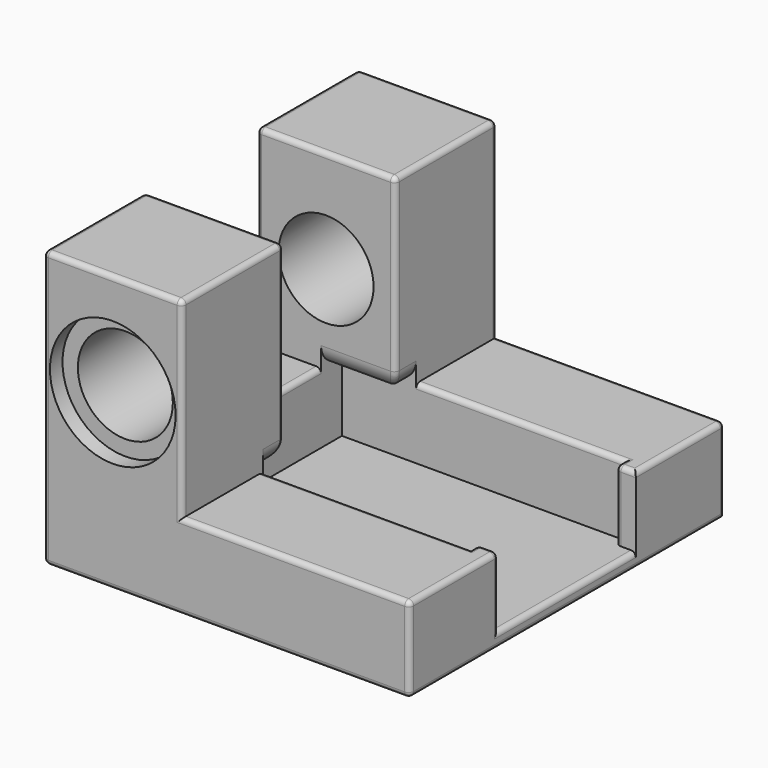
from build123d import *

# Parameters (mm, degrees)
F1_DEPTH  = 39.766
F2_R      = 4.8
F3_DEPTH  = 39.767
F2_R_2    = 6.35
F4_DEPTH  = 1.5875
F5_R      = 6.35
F6_DEPTH  = 1.5875
F7_W      = 7.5
F7_H      = 19.36
F8_DEPTH  = 7.1
F10_DEPTH = 19.3
F11_R     = 2
F12_R     = 0.5


with BuildPart() as f1:
    # F0 (on Front) → F1 (new body)
    with BuildSketch(Plane.XZ):
        Polygon((0, 27.9), (0, 0), (37, 0), (37, 8.6), (14, 8.6), (14, 27.9), align=None)
    extrude(amount=F1_DEPTH)

    # F2 (on face) → F3 (cut, through all)
    with BuildSketch(Plane.XZ.offset(39.766)):
        with Locations((7, 17.55)):
            Circle(F2_R)
    extrude(amount=-F3_DEPTH, mode=Mode.SUBTRACT)

    # F2 (on face) → F4 (cut)
    with BuildSketch(Plane.XZ.offset(39.766)):
        with Locations((7, 17.55)):
            Circle(F2_R_2)
        with Locations((7, 17.55)):
            Circle(F2_R, mode=Mode.SUBTRACT)
    extrude(amount=-F4_DEPTH, mode=Mode.SUBTRACT)

    # F5 (on face) → F6 (cut)
    with BuildSketch(Plane.XZ):
        with Locations((7, 17.55)):
            Circle(F5_R)
    extrude(amount=F6_DEPTH, mode=Mode.SUBTRACT)

    # F7 (on face) → F8 (cut)
    with BuildSketch(Plane.XY.offset(8.6)):
        with Locations((10.25, -19.883)):
            Rectangle(F7_W, F7_H)
        Polygon((37, -28.563), (37, -11.203), (35, -11.203), (35, -10.203), (14, -10.203), (14, -29.563), (35, -29.563), (35, -28.563), align=None)
    extrude(amount=-F8_DEPTH, mode=Mode.SUBTRACT)

    # F9 (on face) → F10 (cut, through all)
    with BuildSketch(Plane.XY.offset(27.9)):
        Polygon((0, -12.827), (0, -19.883), (0, -26.939), (14, -26.939), (14, -12.827), align=None)
    extrude(amount=-F10_DEPTH, mode=Mode.SUBTRACT)

    # F11
    f11_edges = [f1.edges().sort_by_distance(p)[0] for p in [
        (10.25, -26.939, 8.6),
        (14, -11.515, 8.6),
        (10.25, -12.827, 8.6),
        (14, -28.251, 8.6),
    ]]
    fillet(f11_edges, radius=F11_R)

    # F12
    f12_edges = [f1.edges().sort_by_distance(p)[0] for p in [
        (24.5, -10.203, 8.6),
        (24.5, -29.563, 8.6),
        (6.5, -19.883, 8.6),
        (37, -5.6015, 8.6),
        (37, -34.1645, 8.6),
        (37, -28.563, 5.05),
        (35, -11.203, 5.05),
        (37, -19.883, 1.5),
        (35, -29.063, 8.6),
        (35, -28.563, 5.05),
        (36, -28.563, 8.6),
        (36, -11.203, 8.6),
        (35, -10.703, 8.6),
        (25.5, 0, 8.6),
        (25.5, -39.766, 8.6),
        (14, -33.3525, 27.9),
        (7, -26.939, 27.9),
        (0, -33.3525, 27.9),
        (7, -39.766, 27.9),
        (7, -12.827, 27.9),
        (0, -19.883, 8.6),
        (0, -6.4135, 27.9),
        (7, 0, 27.9),
        (14, -6.4135, 27.9),
        (14, -12.827, 19.25),
        (0, -12.827, 18.25),
        (0, 0, 13.95),
        (0, -19.883, 0),
        (0, -39.766, 13.95),
        (14, -39.766, 18.25),
        (14, -26.939, 19.25),
        (14, 0, 18.25),
        (18.5, -39.766, 0),
        (37, -19.883, 0),
        (37, -39.766, 4.3),
        (37, 0, 4.3),
        (0, -26.939, 18.25),
        (13.414214, -12.241214, 9.185786),
        (13.414214, -27.524786, 9.185786),
    ]]
    fillet(f12_edges, radius=F12_R)


solid = f1.part
